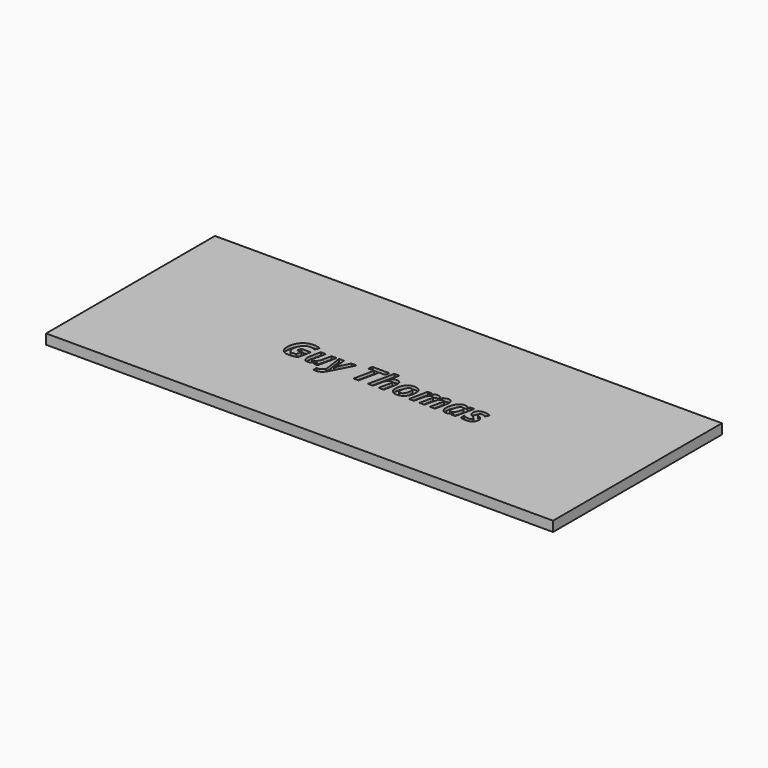
from build123d import *

# Parameters (mm, degrees)
F0_W         = 128.6953315139
F0_H         = 53.5916052759
F1_DEPTH     = 2.54
F2_TEXT_SIZE = 8.74378076
F3_DEPTH     = 0.762


# Not quite as in the source:
# - Text() gives the source's letters only with a copy of the font that has no kerning and outlines rounded to 1/6400 em; it was checked with that copy


with BuildPart() as f1:
    # F0 (on Top) → F1 (new body)
    with BuildSketch(Plane.XY):
        with Locations((1.6983263195, -2.4531371891)):
            Rectangle(F0_W, F0_H)
    extrude(amount=F1_DEPTH)

    # F2 (on face) → F3 (cut)
    with BuildSketch(Plane.XY.offset(2.54)):
        with Locations((-22.2394099803, -6.2955221472)):
            Text('Guy Thomas', F2_TEXT_SIZE, font='Open Sans', font_style=FontStyle.BOLDITALIC, text_align=(TextAlign.LEFT, TextAlign.BOTTOM))
    extrude(amount=-F3_DEPTH, mode=Mode.SUBTRACT)


solid = f1.part
